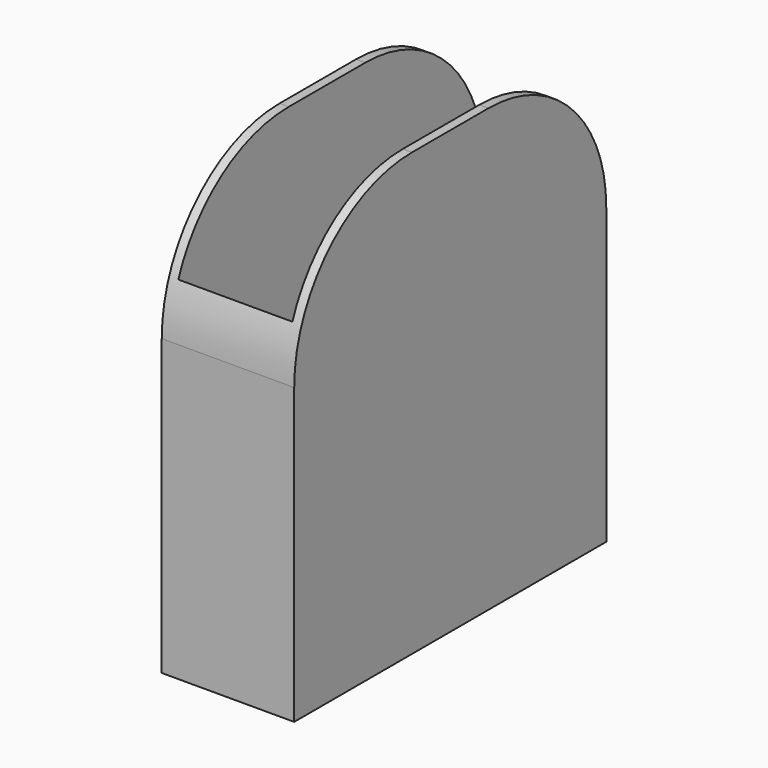
from build123d import *

# Parameters (mm, degrees)
F1_DEPTH    = 1.8
F0_W        = 7.2
F0_H        = 21.2
F2_DEPTH    = 24
F3_T1_DEPTH = 47.2


# Not quite as in the source:
# - a fillet or chamfer that OpenCascade refuses, or shapes differently, is made with other operations: its cross-section is extruded or revolved along the edge and cut away or added


with BuildPart() as f1:
    # F0 (on Top) → F1 (new body)
    with BuildSketch(Plane.XY):
        Polygon((0, 7.1), (0, 0), (6.2, 0), (6.2, 20.2), (0, 20.2), (0, 13.1), (3, 13.1), (3, 10.1), (3, 7.1), align=None)
    extrude(amount=F1_DEPTH)

    # F0 (on Top) → F2 (join)
    with BuildSketch(Plane.XY):
        with Locations((3.1, 10.1)):
            Rectangle(F0_W, F0_H)
        Polygon((6.2, 0), (0, 0), (0, 7.1), (0, 10.1), (0, 13.1), (0, 20.2), (6.2, 20.2), align=None, mode=Mode.SUBTRACT)
    extrude(amount=F2_DEPTH)

    # F3: fillet of radius 8 on 2 edges, made by hand

    # F3_s2 → F3_t1 (cut)
    with BuildSketch(Plane.YZ.offset(-20.5)):
        with BuildLine():
            ThreePointArc((7.5, 24), (1.8431457505, 21.6568542495), (-0.5, 16))
            Line((-0.5, 16), (-0.5, 24))
            Line((-0.5, 24), (7.5, 24))
        make_face()
        with BuildLine():
            ThreePointArc((12.7, 24), (18.3568542495, 21.6568542495), (20.7, 16))
            Line((20.7, 16), (20.7, 24))
            Line((20.7, 24), (12.7, 24))
        make_face()
    extrude(amount=F3_T1_DEPTH, mode=Mode.SUBTRACT)


solid = f1.part
